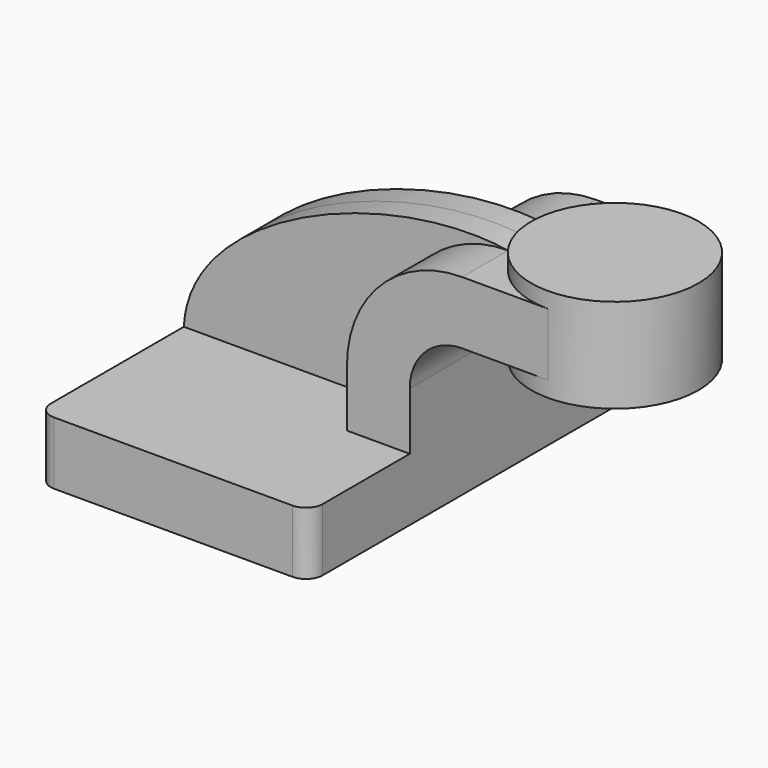
from build123d import *

# Parameters (mm, degrees)
F1_DEPTH = 63.5
F2_DEPTH = 25.4
F3_DEPTH = 7.9375
F5_R     = 5.08


# Not quite as in the source:
# - ends of sketch curves that miss each other by under 0.0002 mm in the source are joined


with BuildPart() as f1:
    # F0 (on Front) → F1 (new body, symmetric)
    with BuildSketch(Plane.XZ):
        Polygon((41.275, -9.525), (41.275, 9.525), (22.225, 9.525), (-41.275, 9.525), (-41.275, -9.525), align=None)
    extrude(amount=F1_DEPTH, both=True)

    # F0 (on Front) → F2 (join, symmetric)
    with BuildSketch(Plane.XZ):
        with BuildLine():
            Line((22.225, 9.525), (41.275, 9.525))
            Line((41.275, 9.525), (41.275, 27.0002))
            ThreePointArc((41.275, 27.0002), (45.9246798487, 38.2255201513), (57.15, 42.8752))
            Line((57.15, 42.8752), (57.8334331512, 42.8752))
            Line((57.8334331512, 42.8752), (57.8334331512, 61.9252))
            Line((57.8334331512, 61.9252), (57.15, 61.9252))
            ThreePointArc((57.15, 61.9252), (32.4542956671, 51.6959043329), (22.225, 27.0002))
            Line((22.225, 27.0002), (22.225, 9.525))
        make_face()
        Polygon((57.8334331512, 61.9252), (57.8334331512, 42.8752), (83.2334309816, 42.8752), (83.2334331512, 61.9252), align=None)
    extrude(amount=F2_DEPTH, both=True)

    # F0 (on Front) → F3 (join, symmetric)
    with BuildSketch(Plane.XZ):
        with BuildLine():
            Line((-41.275, 9.525), (22.225, 9.525))
            Line((22.225, 9.525), (22.225, 27.0002))
            ThreePointArc((22.225, 27.0002), (32.4542956671, 51.6959043329), (57.15, 61.9252))
            add(Edge.make_bspline(
                [(-41.275, 9.525), (-39.7025756538, 42.9233573377), (20.2414225787, 67.5613582134), (57.15, 61.9252)],
                knots=[0, 0, 0, 0, 111.5045361635, 111.5045361635, 111.5045361635, 111.5045361635], degree=3))
        make_face()
    extrude(amount=F3_DEPTH, both=True)

    # F0 (on Front) → F4 (revolve)
    with BuildSketch(Plane.XZ):
        Polygon((83.2334331512, 61.9252), (83.2334331512, 42.8752), (83.2334331512, 38.1), (108.6334331512, 38.1), (108.6334331512, 66.675), (83.2334331512, 66.675), align=None)
    revolve(axis=Axis((83.2334331512, 0, 52.3875), (0, 0, 1)))

    # F5
    f5_edges = [f1.edges().sort_by_distance(p)[0] for p in [
        (-41.275, -63.5, 0),
        (41.275, -63.5, 0),
        (-41.275, 63.5, 0),
        (41.275, 63.5, 0),
    ]]
    fillet(f5_edges, radius=F5_R)


solid = f1.part
